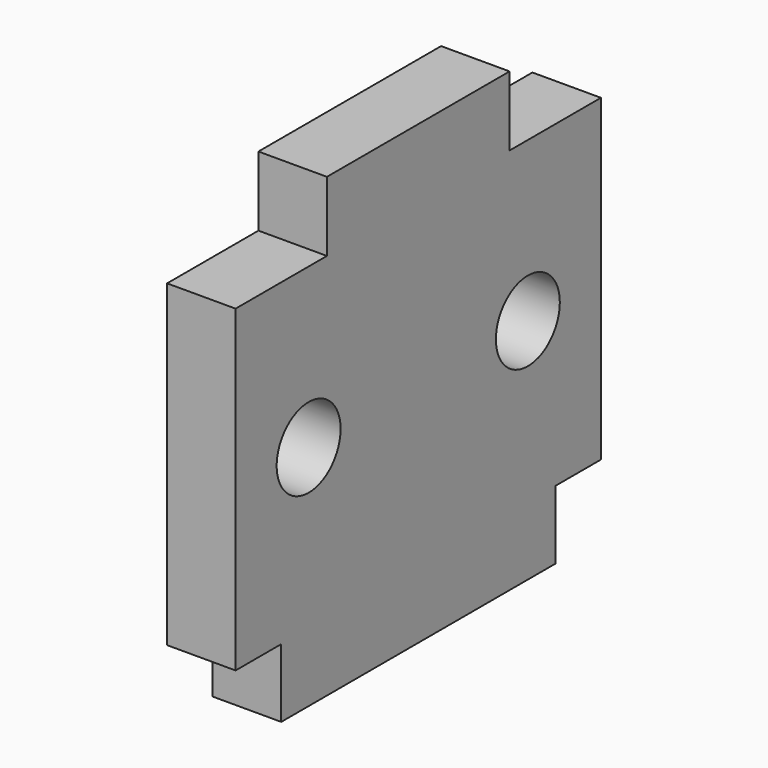
from build123d import *

# Parameters (mm, degrees)
F0_W     = 15
F0_H     = 3
F0_R     = 1.75
F0_W_2   = 10
F0_H_2   = 3.05
F1_DEPTH = 3


# Not quite as in the source:
# - a feature names something its author has since deleted; it is built from what else it names


with BuildPart() as f1:
    # F0 (on Right) → F1 (new body)
    with BuildSketch(Plane.YZ):
        with Locations((0, -8.475)):
            Rectangle(F0_W, F0_H)
        Polygon((7.5, -6.975), (10, -6.975), (10, 6.975), (5, 6.975), (-5, 6.975), (-10, 6.975), (-10, -6.975), (-7.5, -6.975), align=None)
        with Locations((-6, 0)):
            Circle(F0_R, mode=Mode.SUBTRACT)
        with Locations((6, 0)):
            Circle(F0_R, mode=Mode.SUBTRACT)
        with Locations((0, 8.5)):
            Rectangle(F0_W_2, F0_H_2)
    extrude(amount=F1_DEPTH)


solid = f1.part
